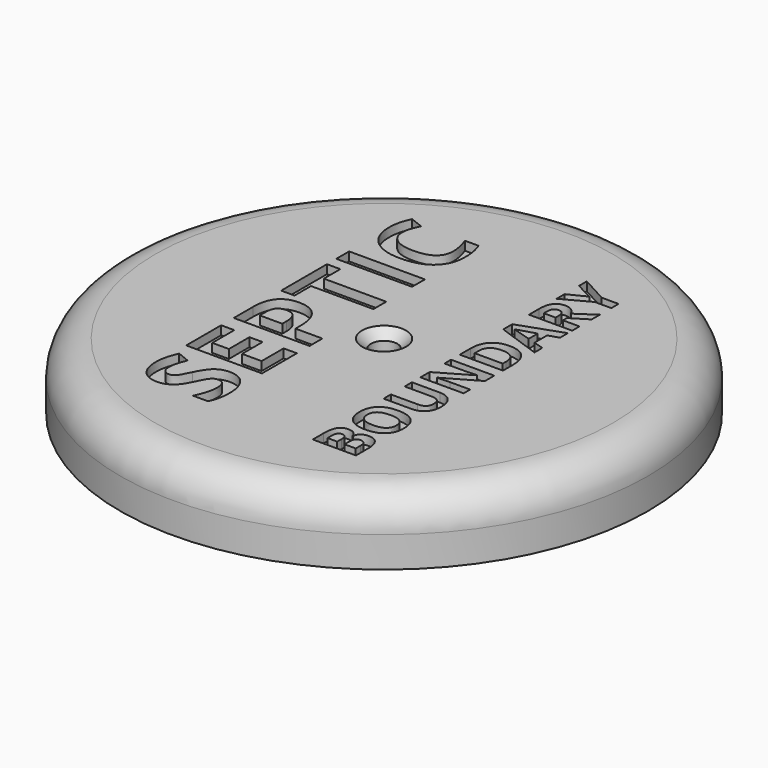
from build123d import *

# Parameters (mm, degrees)
F0_R           = 38.1
F1_DEPTH       = 9.525
F3_R           = 5.08
F4_TEXT_SIZE   = 15.3206729183
F4_TEXT_SIZE_2 = 8.7343846546
F5_DEPTH       = 1.27
F2_R           = 1.905
F6_DEPTH       = 25.4
F7_SIZE        = 1.27


# Not quite as in the source:
# - Text() gives the source's letters only with a copy of the font that has no kerning and outlines rounded to 1/6400 em; it was checked with that copy


with BuildPart() as f1:
    # F0 (on Top) → F1 (new body)
    with BuildSketch(Plane.XY):
        Circle(F0_R)
    extrude(amount=F1_DEPTH)

    # F3
    f3_edges = [f1.edges().sort_by_distance(p)[0] for p in [
        (-38.1, 0, 9.525),
    ]]
    fillet(f3_edges, radius=F3_R)

    # F4 (on face) → F5 (cut)
    with BuildSketch(Plane.XY.offset(9.525)):
        with Locations(Location((-5.4390758838, -25.0442931811), (0, 0, 90))):
            Text('SEPTIC', F4_TEXT_SIZE, font='Open Sans', font_style=FontStyle.BOLD, text_align=(TextAlign.LEFT, TextAlign.BOTTOM))
        with Locations(Location((15.3447269797, -25.0393819898), (0, 0, 90))):
            Text('BOUNDARY', F4_TEXT_SIZE_2, font='Open Sans', font_style=FontStyle.BOLD, text_align=(TextAlign.LEFT, TextAlign.BOTTOM))
    extrude(amount=-F5_DEPTH, mode=Mode.SUBTRACT)

    # F2 (on face) → F6 (cut)
    with BuildSketch(Plane(origin=(0, 0, 0), x_dir=(1, 0, 0), z_dir=(0, 0, -1))):
        Circle(F2_R)
    extrude(amount=-F6_DEPTH, mode=Mode.SUBTRACT)

    # F7
    f7_edges = [f1.edges().sort_by_distance(p)[0] for p in [
        (-1.905, 0, 9.525),
    ]]
    chamfer(f7_edges, length=F7_SIZE)


solid = f1.part
